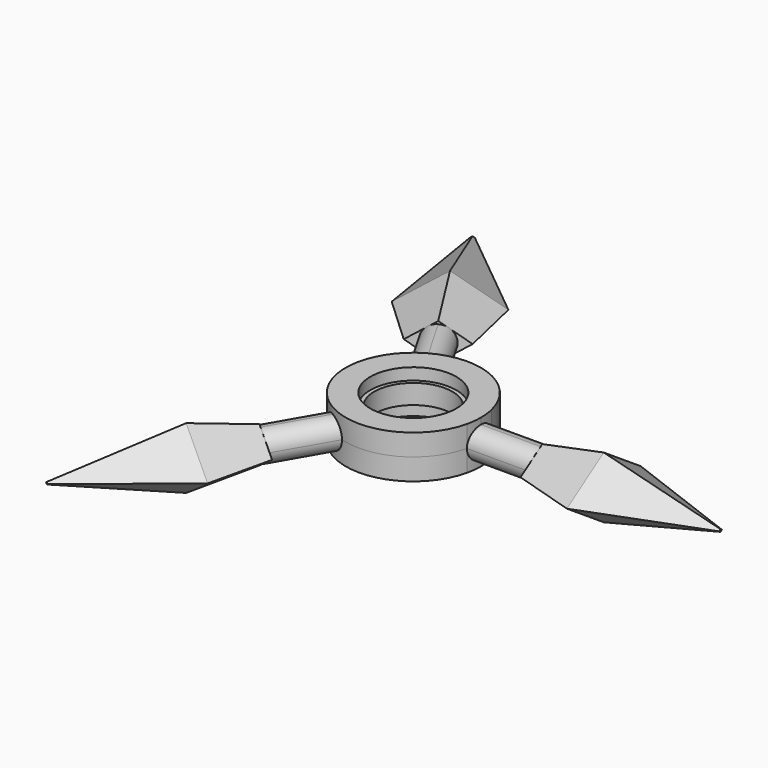
from build123d import *

# Parameters (mm, degrees)
F0_R         = 7
F1_DEPTH     = 3.5
F2_DEPTH     = 5
F3_SIZE2     = 7.49999
F3_SIZE      = 4.99999
F3_2_SIZE2   = 7.49999
F3_2_SIZE    = 4.99999
F4_SIZE2     = 19
F4_SIZE      = 4
F5_T1_DEPTH  = 51.9728125874
F5_T3_DEPTH  = 60.9866569086
F5_T5_DEPTH  = 60.9866569086
F5_T7_DEPTH  = 51.9728125874
F5_T9_DEPTH  = 60.9866569086
F5_T11_DEPTH = 60.9866569086
F5_T16_DEPTH = 61.9841307208
F5_T21_DEPTH = 61.9841307208
F5_T26_DEPTH = 61.9841307208
F5_T31_DEPTH = 61.9841307208
F5_T36_DEPTH = 61.9934705111
F5_T41_DEPTH = 61.9934705111
F5_T46_DEPTH = 61.9934705111
F5_T51_DEPTH = 61.9934705111
F5_T56_DEPTH = 61.9934705111
F5_T61_DEPTH = 61.9934705111
F5_T66_DEPTH = 61.9934705111
F5_T71_DEPTH = 61.9934705111
F5_T76_DEPTH = 61.9841307208
F5_T81_DEPTH = 61.9841307208
F5_T86_DEPTH = 61.9841307208
F5_T91_DEPTH = 61.9841307208
F6_DEPTH     = 2.5
F7_R         = 2.4999
F8_COUNT     = 3
F0_R_2       = 6.35
F9_DEPTH     = 1.5875


# Not quite as in the source:
# - a fillet or chamfer that OpenCascade refuses, or shapes differently, is made with other operations: its cross-section is extruded or revolved along the edge and cut away or added
# - a fillet or chamfer is up to 0.001 mm smaller than in the source, because OpenCascade refuses the exact size


with BuildPart() as f1:
    # F0 (on Top) → F1 (new body, symmetric)
    with BuildSketch(Plane.XY):
        with BuildLine():
            Line((10.7121426428, -2.5), (10.7121426428, 2.5))
            ThreePointArc((10.7121426428, 2.5), (-11, 0), (10.7121426428, -2.5))
        make_face()
        Circle(F0_R, mode=Mode.SUBTRACT)
        with BuildLine():
            ThreePointArc((10.7121426428, -2.5), (10.9277987049, -1.258258902), (11, 0))
            ThreePointArc((11, 0), (10.9277987049, 1.258258902), (10.7121426428, 2.5))
            Line((10.7121426428, 2.5), (10.7121426428, -2.5))
        make_face()
    extrude(amount=F1_DEPTH, both=True)

    # F0 (on Top) → F9 (join, symmetric)
    with BuildSketch(Plane.XY):
        Circle(F0_R)
        Circle(F0_R_2, mode=Mode.SUBTRACT)
    extrude(amount=F9_DEPTH, both=True)


with BuildPart() as f2:
    # F0 (on Top) → F2 (new body, symmetric)
    with BuildSketch(Plane.XY):
        Polygon((31, 7.5), (21, 2.5), (21, -2.5), (31, -7.5), (50, 0), align=None)
        Polygon((21, 7.5), (21, 2.5), (31, 7.5), align=None)
        Polygon((31, -7.5), (21, -2.5), (21, -7.5), align=None)
        Polygon((50, 7.5), (31, 7.5), (50, 0), align=None)
        Polygon((50, 0), (31, -7.5), (50, -7.5), align=None)
    extrude(amount=F2_DEPTH, both=True)

    # F3 (size 5 and 7.5 in the source; OpenCascade refuses exactly that, so slightly less here)
    f3_edges = [f2.edges().sort_by_distance(p)[0] for p in [
        (35.5, 7.5, 5),
        (35.5, 7.5, -5),
    ]]
    f3_side = f2.faces().sort_by_distance((35.5, 7.5, 0))[0]
    chamfer(f3_edges, length=F3_SIZE, length2=F3_SIZE2, reference=f3_side)

    # F3#2 (size 5 and 7.5 in the source; OpenCascade refuses exactly that, so slightly less here)
    f3_2_edges = [f2.edges().sort_by_distance(p)[0] for p in [
        (35.5, -7.5, 5),
        (35.5, -7.5, -5),
    ]]
    f3_2_side = f2.faces().sort_by_distance((35.5, -7.5, 0))[0]
    chamfer(f3_2_edges, length=F3_2_SIZE, length2=F3_2_SIZE2, reference=f3_2_side)

    # F4 (call 1 of 4: OpenCascade refuses the feature's edges together)
    f4_edges = [f2.edges().sort_by_distance(p)[0] for p in [
        (50, 3.750005, 2.500005),
    ]]
    f4_side = f2.faces().sort_by_distance((50, 0, 0))[0]
    chamfer(f4_edges, length=F4_SIZE, length2=F4_SIZE2, reference=f4_side)

    # F4#2 (call 2 of 4)
    f4_2_edges = [f2.edges().sort_by_distance(p)[0] for p in [
        (50, -3.750005, 2.500005),
    ]]
    f4_2_side = f2.faces().sort_by_distance((50, 0, 0))[0]
    chamfer(f4_2_edges, length=F4_SIZE, length2=F4_SIZE2, reference=f4_2_side)

    # F4#3 (call 3 of 4)
    f4_3_edges = [f2.edges().sort_by_distance(p)[0] for p in [
        (50, -3.750005, -2.500005),
    ]]
    f4_3_side = f2.faces().sort_by_distance((50, 0, 0))[0]
    chamfer(f4_3_edges, length=F4_SIZE, length2=F4_SIZE2, reference=f4_3_side)

    # F4#4 (call 4 of 4)
    f4_4_edges = [f2.edges().sort_by_distance(p)[0] for p in [
        (50, 3.750005, -2.500005),
    ]]
    f4_4_side = f2.faces().sort_by_distance((50, 0, 0))[0]
    chamfer(f4_4_edges, length=F4_SIZE, length2=F4_SIZE2, reference=f4_4_side)

    # F5: chamfer of 1.7 x 10 on 16 edges, made by hand

    # F5_s2 → F5_t1 (cut)
    with BuildSketch(Plane.XY.offset(-25.9864062937)):
        Polygon((31, 7.5), (21, 5.8), (21, 7.5), align=None)
        Polygon((31, -7.5), (21, -5.8), (21, -7.5), align=None)
    extrude(amount=F5_T1_DEPTH, mode=Mode.SUBTRACT)

    # F5_s4 → F5_t3 (cut)
    with BuildSketch(Plane(origin=(0, 26.8142983273, 17.8761869674), x_dir=(1, 0, 0), z_dir=(0, -0.832050465, -0.5546999402))):
        Polygon((31, -4.1602578721), (21, -2.4602578721), (21, -4.1602578721), align=None)
    extrude(amount=F5_T3_DEPTH, mode=Mode.SUBTRACT)

    # F5_s6 → F5_t5 (cut)
    with BuildSketch(Plane(origin=(0, 26.8142983273, -17.8761869674), x_dir=(1, 0, 0), z_dir=(0, -0.832050465, 0.5546999402))):
        Polygon((31, 4.1602578721), (21, 2.4602578721), (21, 4.1602578721), align=None)
    extrude(amount=F5_T5_DEPTH, mode=Mode.SUBTRACT)

    # F5_s8 → F5_t7 (cut)
    with BuildSketch(Plane.XZ.offset(-25.9864062937)):
        Polygon((31, -5), (21, -3.3), (21, -5), align=None)
        Polygon((31, 5), (21, 3.3), (21, 5), align=None)
    extrude(amount=F5_T7_DEPTH, mode=Mode.SUBTRACT)

    # F5_s10 → F5_t9 (cut)
    with BuildSketch(Plane(origin=(0, -26.8142983273, 17.8761869674), x_dir=(1, 0, 0), z_dir=(0, 0.832050465, -0.5546999402))):
        Polygon((31, 4.1602578721), (21, 2.4602578721), (21, 4.1602578721), align=None)
    extrude(amount=F5_T9_DEPTH, mode=Mode.SUBTRACT)

    # F5_s12 → F5_t11 (cut)
    with BuildSketch(Plane(origin=(0, -26.8142983273, -17.8761869674), x_dir=(1, 0, 0), z_dir=(0, 0.832050465, 0.5546999402))):
        Polygon((31, -4.1602578721), (21, -2.4602578721), (21, -4.1602578721), align=None)
    extrude(amount=F5_T11_DEPTH, mode=Mode.SUBTRACT)


with BuildPart() as f5_tool14:
    # F5_s15 → F5_t16 (new body)
    with BuildSketch(Plane.YZ.offset(56.9920653604)):
        Polygon((7.5, 1.69999), (-0.8205046502, -5.5470094021), (7.5, -1e-05), align=None)
    extrude(amount=-F5_T16_DEPTH)

    split(bisect_by=Plane(origin=(0.1833571404, -0.5982834989, 0.8974258466), x_dir=(-0.9561063641, -0.2930198295, 0), z_dir=(-0.1675954939, 0.5468541792, -0.8202818157)), keep=Keep.TOP)


with BuildPart() as f2_1:
    add(f2.part)

    # F5_t13: cut F5_tool14
    add(f5_tool14.part, mode=Mode.SUBTRACT)


with BuildPart() as f5_tool19:
    # F5_s20 → F5_t21 (new body)
    with BuildSketch(Plane.YZ.offset(56.9920653604)):
        Polygon((7.5, 1.69999), (-0.8205046502, -5.5470094021), (7.5, -1e-05), align=None)
    extrude(amount=-F5_T21_DEPTH)

    split(bisect_by=Plane(origin=(-0.3684517446, 2.1673632034, 0), x_dir=(0, 0, 1), z_dir=(-0.1675954939, 0.9858558467, 0)), keep=Keep.TOP)


with BuildPart() as f2_2:
    add(f2_1.part)

    # F5_t18: cut F5_tool19
    add(f5_tool19.part, mode=Mode.SUBTRACT)


with BuildPart() as f5_tool24:
    # F5_s25 → F5_t26 (new body)
    with BuildSketch(Plane.YZ.offset(56.9920653604)):
        Polygon((7.5, -1.69999), (-0.8205046502, 5.5470094021), (7.5, 1e-05), align=None)
    extrude(amount=-F5_T26_DEPTH)

    split(bisect_by=Plane(origin=(0.1833571404, -0.5982834989, -0.8974258466), x_dir=(-0.9561063641, -0.2930198295, 0), z_dir=(-0.1675954939, 0.5468541792, 0.8202818157)), keep=Keep.TOP)


with BuildPart() as f2_3:
    add(f2_2.part)

    # F5_t23: cut F5_tool24
    add(f5_tool24.part, mode=Mode.SUBTRACT)


with BuildPart() as f5_tool29:
    # F5_s30 → F5_t31 (new body)
    with BuildSketch(Plane.YZ.offset(56.9920653604)):
        Polygon((7.5, -1.69999), (-0.8205046502, 5.5470094021), (7.5, 1e-05), align=None)
    extrude(amount=-F5_T31_DEPTH)

    split(bisect_by=Plane(origin=(-0.3684517446, 2.1673632034, 0), x_dir=(0, 0, 1), z_dir=(-0.1675954939, 0.9858558467, 0)), keep=Keep.TOP)


with BuildPart() as f2_4:
    add(f2_3.part)

    # F5_t28: cut F5_tool29
    add(f5_tool29.part, mode=Mode.SUBTRACT)


with BuildPart() as f5_tool34:
    # F5_s35 → F5_t36 (new body)
    with BuildSketch(Plane.YZ.offset(-4.9967352555)):
        Polygon((1.69999, -5), (-8.3205146502, 0.5469994021), (-1e-05, -5), align=None)
    extrude(amount=F5_T36_DEPTH)

    split(bisect_by=Plane(origin=(0.0446107493, 0, 0.2624161726), x_dir=(0, 1, 0), z_dir=(-0.1675954939, 0, -0.9858558467)), keep=Keep.TOP)


with BuildPart() as f2_5:
    add(f2_4.part)

    # F5_t33: cut F5_tool34
    add(f5_tool34.part, mode=Mode.SUBTRACT)


with BuildPart() as f5_tool39:
    # F5_s40 → F5_t41 (new body)
    with BuildSketch(Plane.YZ.offset(-4.9967352555)):
        Polygon((1.69999, -5), (-8.3205146502, 0.5469994021), (-1e-05, -5), align=None)
    extrude(amount=F5_T41_DEPTH)

    split(bisect_by=Plane(origin=(0.1833571404, 0.5982834989, 0.8974258466), x_dir=(0.9561063641, -0.2930198295, 0), z_dir=(-0.1675954939, -0.5468541792, -0.8202818157)), keep=Keep.TOP)


with BuildPart() as f2_6:
    add(f2_5.part)

    # F5_t38: cut F5_tool39
    add(f5_tool39.part, mode=Mode.SUBTRACT)


with BuildPart() as f5_tool44:
    # F5_s45 → F5_t46 (new body)
    with BuildSketch(Plane.YZ.offset(56.9967352555)):
        Polygon((-1.69999, -5), (8.3205146502, 0.5469994021), (1e-05, -5), align=None)
    extrude(amount=-F5_T46_DEPTH)

    split(bisect_by=Plane(origin=(0.1833571404, -0.5982834989, 0.8974258466), x_dir=(-0.9561063641, -0.2930198295, 0), z_dir=(-0.1675954939, 0.5468541792, -0.8202818157)), keep=Keep.TOP)


with BuildPart() as f2_7:
    add(f2_6.part)

    # F5_t43: cut F5_tool44
    add(f5_tool44.part, mode=Mode.SUBTRACT)


with BuildPart() as f5_tool49:
    # F5_s50 → F5_t51 (new body)
    with BuildSketch(Plane.YZ.offset(56.9967352555)):
        Polygon((-1.69999, -5), (8.3205146502, 0.5469994021), (1e-05, -5), align=None)
    extrude(amount=-F5_T51_DEPTH)

    split(bisect_by=Plane(origin=(0.0446107493, 0, 0.2624161726), x_dir=(0, 1, 0), z_dir=(-0.1675954939, 0, -0.9858558467)), keep=Keep.TOP)


with BuildPart() as f2_8:
    add(f2_7.part)

    # F5_t48: cut F5_tool49
    add(f5_tool49.part, mode=Mode.SUBTRACT)


with BuildPart() as f5_tool54:
    # F5_s55 → F5_t56 (new body)
    with BuildSketch(Plane.YZ.offset(-4.9967352555)):
        Polygon((1.69999, 5), (-8.3205146502, -0.5469994021), (-1e-05, 5), align=None)
    extrude(amount=F5_T56_DEPTH)

    split(bisect_by=Plane(origin=(0.1833571404, 0.5982834989, -0.8974258466), x_dir=(0.9561063641, -0.2930198295, 0), z_dir=(-0.1675954939, -0.5468541792, 0.8202818157)), keep=Keep.TOP)


with BuildPart() as f2_9:
    add(f2_8.part)

    # F5_t53: cut F5_tool54
    add(f5_tool54.part, mode=Mode.SUBTRACT)


with BuildPart() as f5_tool59:
    # F5_s60 → F5_t61 (new body)
    with BuildSketch(Plane.YZ.offset(-4.9967352555)):
        Polygon((1.69999, 5), (-8.3205146502, -0.5469994021), (-1e-05, 5), align=None)
    extrude(amount=F5_T61_DEPTH)

    split(bisect_by=Plane(origin=(0.0446107493, 0, -0.2624161726), x_dir=(0, 1, 0), z_dir=(-0.1675954939, 0, 0.9858558467)), keep=Keep.TOP)


with BuildPart() as f2_10:
    add(f2_9.part)

    # F5_t58: cut F5_tool59
    add(f5_tool59.part, mode=Mode.SUBTRACT)


with BuildPart() as f5_tool64:
    # F5_s65 → F5_t66 (new body)
    with BuildSketch(Plane.YZ.offset(56.9967352555)):
        Polygon((-1.69999, 5), (8.3205146502, -0.5469994021), (1e-05, 5), align=None)
    extrude(amount=-F5_T66_DEPTH)

    split(bisect_by=Plane(origin=(0.1833571404, -0.5982834989, -0.8974258466), x_dir=(-0.9561063641, -0.2930198295, 0), z_dir=(-0.1675954939, 0.5468541792, 0.8202818157)), keep=Keep.TOP)


with BuildPart() as f2_11:
    add(f2_10.part)

    # F5_t63: cut F5_tool64
    add(f5_tool64.part, mode=Mode.SUBTRACT)


with BuildPart() as f5_tool69:
    # F5_s70 → F5_t71 (new body)
    with BuildSketch(Plane.YZ.offset(56.9967352555)):
        Polygon((-1.69999, 5), (8.3205146502, -0.5469994021), (1e-05, 5), align=None)
    extrude(amount=-F5_T71_DEPTH)

    split(bisect_by=Plane(origin=(0.0446107493, 0, -0.2624161726), x_dir=(0, 1, 0), z_dir=(-0.1675954939, 0, 0.9858558467)), keep=Keep.TOP)


with BuildPart() as f2_12:
    add(f2_11.part)

    # F5_t68: cut F5_tool69
    add(f5_tool69.part, mode=Mode.SUBTRACT)


with BuildPart() as f5_tool74:
    # F5_s75 → F5_t76 (new body)
    with BuildSketch(Plane.YZ.offset(-4.9920653604)):
        Polygon((-7.5, 1.69999), (0.8205046502, -5.5470094021), (-7.5, -1e-05), align=None)
    extrude(amount=F5_T76_DEPTH)

    split(bisect_by=Plane(origin=(0.1833571404, 0.5982834989, 0.8974258466), x_dir=(0.9561063641, -0.2930198295, 0), z_dir=(-0.1675954939, -0.5468541792, -0.8202818157)), keep=Keep.TOP)


with BuildPart() as f2_13:
    add(f2_12.part)

    # F5_t73: cut F5_tool74
    add(f5_tool74.part, mode=Mode.SUBTRACT)


with BuildPart() as f5_tool79:
    # F5_s80 → F5_t81 (new body)
    with BuildSketch(Plane.YZ.offset(-4.9920653604)):
        Polygon((-7.5, 1.69999), (0.8205046502, -5.5470094021), (-7.5, -1e-05), align=None)
    extrude(amount=F5_T81_DEPTH)

    split(bisect_by=Plane(origin=(-0.3684517446, -2.1673632034, 0), x_dir=(0, 0, 1), z_dir=(-0.1675954939, -0.9858558467, 0)), keep=Keep.TOP)


with BuildPart() as f2_14:
    add(f2_13.part)

    # F5_t78: cut F5_tool79
    add(f5_tool79.part, mode=Mode.SUBTRACT)


with BuildPart() as f5_tool84:
    # F5_s85 → F5_t86 (new body)
    with BuildSketch(Plane.YZ.offset(-4.9920653604)):
        Polygon((-7.5, -1.69999), (0.8205046502, 5.5470094021), (-7.5, 1e-05), align=None)
    extrude(amount=F5_T86_DEPTH)

    split(bisect_by=Plane(origin=(0.1833571404, 0.5982834989, -0.8974258466), x_dir=(0.9561063641, -0.2930198295, 0), z_dir=(-0.1675954939, -0.5468541792, 0.8202818157)), keep=Keep.TOP)


with BuildPart() as f2_15:
    add(f2_14.part)

    # F5_t83: cut F5_tool84
    add(f5_tool84.part, mode=Mode.SUBTRACT)


with BuildPart() as f5_tool89:
    # F5_s90 → F5_t91 (new body)
    with BuildSketch(Plane.YZ.offset(-4.9920653604)):
        Polygon((-7.5, -1.69999), (0.8205046502, 5.5470094021), (-7.5, 1e-05), align=None)
    extrude(amount=F5_T91_DEPTH)

    split(bisect_by=Plane(origin=(-0.3684517446, -2.1673632034, 0), x_dir=(0, 0, 1), z_dir=(-0.1675954939, -0.9858558467, 0)), keep=Keep.TOP)


with BuildPart() as f2_16:
    add(f2_15.part)

    # F5_t88: cut F5_tool89
    add(f5_tool89.part, mode=Mode.SUBTRACT)


with BuildPart() as f6:
    # F0 (on Top) → F6 (new body, symmetric)
    with BuildSketch(Plane.XY):
        with BuildLine():
            ThreePointArc((10.7121426428, 2.5), (10.9277987049, 1.258258902), (11, 0))
            ThreePointArc((11, 0), (10.9277987049, -1.258258902), (10.7121426428, -2.5))
            Line((10.7121426428, -2.5), (21, -2.5))
            Line((21, -2.5), (21, 2.5))
            Line((21, 2.5), (10.7121426428, 2.5))
        make_face()
    extrude(amount=F6_DEPTH, both=True)

    # F7 (radius 2.5 in the source; OpenCascade refuses exactly that, so slightly less here)
    f7_edges = [f6.edges().sort_by_distance(p)[0] for p in [
        (15.856071, -2.5, 2.5),
        (15.856071, 2.5, 2.5),
        (15.856071, -2.5, -2.5),
        (15.856071, 2.5, -2.5),
    ]]
    fillet(f7_edges, radius=F7_R)


with BuildPart() as f8_1:
    # F8: instance of F2
    add(f2_16.part.rotate(Axis((0, 0, 0), (0, 0, 1)), 1 * 360 / F8_COUNT))


with BuildPart() as f8_2:
    # F8: instance of F2
    add(f2_16.part.rotate(Axis((0, 0, 0), (0, 0, 1)), 2 * 360 / F8_COUNT))


with BuildPart() as f8_3:
    # F8: instance of F6
    add(f6.part.rotate(Axis((0, 0, 0), (0, 0, 1)), 1 * 360 / F8_COUNT))


with BuildPart() as f8_4:
    # F8: instance of F6
    add(f6.part.rotate(Axis((0, 0, 0), (0, 0, 1)), 2 * 360 / F8_COUNT))


solid = Compound([f1.part, f2_16.part, f6.part, f8_1.part, f8_2.part, f8_3.part, f8_4.part])
